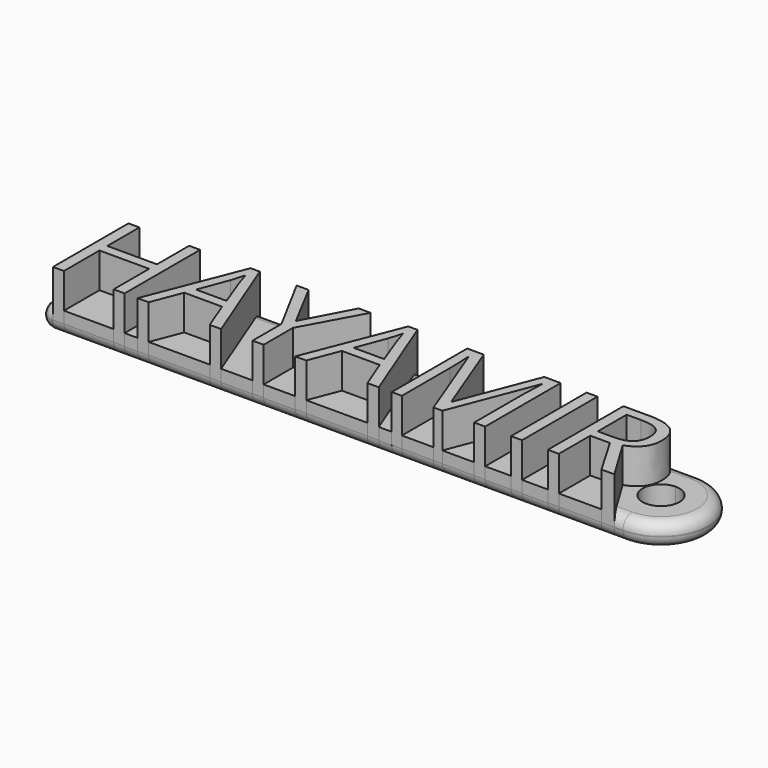
from build123d import *

# Parameters (mm, degrees)
F0_TEXT_SIZE   = 11.3354587318
F1_DEPTH       = 5
F0_W           = 4.2631951824
F0_H           = 3.8080056677
F2_DEPTH       = 2
F3_T1_DEPTH    = 5.9528869996
F3_T3_DEPTH    = 5.9741409848
F3_S1_T1_DEPTH = 5.9511158342
F3_S2_T1_DEPTH = 5.9528869996
F3_S2_T3_DEPTH = 5.9741409848
F3_S3_T1_DEPTH = 5.7580588027
F3_S3_T3_DEPTH = 5.9404888417
F3_S4_T1_DEPTH = 5.6597591215
F3_S5_T1_DEPTH = 5.6597591215
F3_S5_T3_DEPTH = 6.1122918881
F3_S6_T1_DEPTH = 5.9404888417
F3_2_T1_DEPTH  = 9.2631951824
F3_3_T1_DEPTH  = 48.9990343146
F3_3_T3_DEPTH  = 7.2240991066
F3_3_T5_DEPTH  = 7.2240991066
F3_3_T7_DEPTH  = 2.613740616
F3_3_T9_DEPTH  = 6.1118072185
F3_3_T11_DEPTH = 7.7005426064
F3_3_T13_DEPTH = 7.7058561027
F3_3_T15_DEPTH = 6.1595989161
F3_3_T17_DEPTH = 6.1171207148
F3_3_T19_DEPTH = 3.2374480655
F3_3_S23_W     = 1.1015022539
F3_3_S23_H     = 1.101502254
F3_3_T24_DEPTH = 1.101502254
F3_3_S29_W     = 1.1015022539
F3_3_S29_H     = 1.1015022539
F3_3_T30_DEPTH = 1.101502254
F3_3_S35_W     = 1.1015022539
F3_3_S35_H     = 1.1015022539
F3_3_T36_DEPTH = 1.101502254
F3_3_S41_W     = 1.1015022539
F3_3_S41_H     = 1.1015022539
F3_3_T42_DEPTH = 1.101502254
F3_3_T46_ANGLE = 180
F3_3_T48_ANGLE = 180
F3_4_T1_DEPTH  = 8.6486007793
F3_5_T1_DEPTH  = 7.7346794191
F3_6_T1_DEPTH  = 7.7116542685
F3_7_T1_DEPTH  = 10.2461919943
F3_8_T1_DEPTH  = 10.2461919943


# Not quite as in the source:
# - a fillet or chamfer that OpenCascade refuses, or shapes differently, is made with other operations: its cross-section is extruded or revolved along the edge and cut away or added
# - Text() gives the source's letters only with a copy of the font that has no kerning and outlines rounded to 1/6400 em; it was checked with that copy


with BuildPart() as f1:
    # F0 (on Top) → F1 (new body)
    with BuildSketch(Plane.XY):
        with Locations((-50, 0)):
            Text('HAYAMIR', F0_TEXT_SIZE, font='Open Sans', text_align=(TextAlign.LEFT, TextAlign.BOTTOM))
    extrude(amount=F1_DEPTH)

    # F3: fillet of radius 1 on 2 edges, made by hand

    # F3_s2 → F3_t1 (cut)
    with BuildSketch(Plane.YZ.offset(-44.1365568544)):
        with BuildLine():
            ThreePointArc((0, 1), (0.2928932188, 0.2928932188), (1, 0))
            Line((1, 0), (0, 0))
            Line((0, 0), (0, 1))
        make_face()
    extrude(amount=F3_T1_DEPTH, mode=Mode.SUBTRACT)

    # F3_s4 → F3_t3 (cut)
    with BuildSketch(Plane.YZ.offset(-37.9374778604)):
        with BuildLine():
            ThreePointArc((0, 1), (0.2928932188, 0.2928932188), (1, 0))
            Line((1, 0), (0, 0))
            Line((0, 0), (0, 1))
        make_face()
    extrude(amount=F3_T3_DEPTH, mode=Mode.SUBTRACT)

    # F3#s1: fillet of radius 1 on 1 edges, made by hand

    # F3_s1_s2 → F3_s1_t1 (cut)
    with BuildSketch(Plane.YZ.offset(-34.267623096)):
        with BuildLine():
            ThreePointArc((0, 1), (0.2928932188, 0.2928932188), (1, 0))
            Line((1, 0), (0, 0))
            Line((0, 0), (0, 1))
        make_face()
    extrude(amount=F3_S1_T1_DEPTH, mode=Mode.SUBTRACT)

    # F3#s2: fillet of radius 1 on 2 edges, made by hand

    # F3_s2_s2 → F3_s2_t1 (cut)
    with BuildSketch(Plane.YZ.offset(-30.6154799858)):
        with BuildLine():
            ThreePointArc((0, 1), (0.2928932188, 0.2928932188), (1, 0))
            Line((1, 0), (0, 0))
            Line((0, 0), (0, 1))
        make_face()
    extrude(amount=F3_S2_T1_DEPTH, mode=Mode.SUBTRACT)

    # F3_s2_s4 → F3_s2_t3 (cut)
    with BuildSketch(Plane.YZ.offset(-24.4164009919)):
        with BuildLine():
            ThreePointArc((0, 1), (0.2928932188, 0.2928932188), (1, 0))
            Line((1, 0), (0, 0))
            Line((0, 0), (0, 1))
        make_face()
    extrude(amount=F3_S2_T3_DEPTH, mode=Mode.SUBTRACT)

    # F3#s3: fillet of radius 1 on 3 edges, made by hand

    # F3_s3_s2 → F3_s3_t1 (cut)
    with BuildSketch(Plane.YZ.offset(-18.7486716259)):
        with BuildLine():
            ThreePointArc((0, 1), (0.2928932188, 0.2928932188), (1, 0))
            Line((1, 0), (0, 0))
            Line((0, 0), (0, 1))
        make_face()
    extrude(amount=F3_S3_T1_DEPTH, mode=Mode.SUBTRACT)

    # F3_s3_s4 → F3_s3_t3 (cut)
    with BuildSketch(Plane.YZ.offset(-15.2559334042)):
        with BuildLine():
            ThreePointArc((1, 0), (0.2928932188, 0.2928932188), (0, 1))
            Line((0, 1), (0, 0))
            Line((0, 0), (1, 0))
        make_face()
    extrude(amount=F3_S3_T3_DEPTH, mode=Mode.SUBTRACT)

    # F3#s4: fillet of radius 1 on 1 edges, made by hand

    # F3_s4_s2 → F3_s4_t1 (cut)
    with BuildSketch(Plane.YZ.offset(-11.8154445625)):
        with BuildLine():
            ThreePointArc((1, 0), (0.2928932188, 0.2928932188), (0, 1))
            Line((0, 1), (0, 0))
            Line((0, 0), (1, 0))
        make_face()
    extrude(amount=F3_S4_T1_DEPTH, mode=Mode.SUBTRACT)

    # F3#s5: fillet of radius 1 on 2 edges, made by hand

    # F3_s5_s2 → F3_s5_t1 (cut)
    with BuildSketch(Plane.YZ.offset(-8.655685441)):
        with BuildLine():
            ThreePointArc((1, 0), (0.2928932188, 0.2928932188), (0, 1))
            Line((0, 1), (0, 0))
            Line((0, 0), (1, 0))
        make_face()
    extrude(amount=F3_S5_T1_DEPTH, mode=Mode.SUBTRACT)

    # F3_s5_s4 → F3_s5_t3 (cut)
    with BuildSketch(Plane.YZ.offset(-4.3473255402)):
        with BuildLine():
            ThreePointArc((0, 1), (0.2928932188, 0.2928932188), (1, 0))
            Line((1, 0), (0, 0))
            Line((0, 0), (0, 1))
        make_face()
    extrude(amount=F3_S5_T3_DEPTH, mode=Mode.SUBTRACT)

    # F3#s6: fillet of radius 1 on 2 edges, made by hand

    # F3_s6_s2 → F3_s6_t1 (cut)
    with BuildSketch(Plane.YZ.offset(-51.3877081119)):
        with BuildLine():
            ThreePointArc((1, 0), (0.2928932188, 0.2928932188), (0, 1))
            Line((0, 1), (0, 0))
            Line((0, 0), (1, 0))
        make_face()
    extrude(amount=F3_S6_T1_DEPTH, mode=Mode.SUBTRACT)


with BuildPart() as f2:
    # F0 (on Top) → F2 (new body)
    with BuildSketch(Plane.XY):
        with Locations((-45.8156216791, 1.9040028339)):
            Rectangle(F0_W, F0_H)
    extrude(amount=F2_DEPTH)

    # F3#2: fillet of radius 1 on 1 edges, made by hand

    # F3_2_s2 → F3_2_t1 (cut)
    with BuildSketch(Plane.YZ.offset(-50.4472192703)):
        with BuildLine():
            ThreePointArc((0, 1), (0.2928932188, 0.2928932188), (1, 0))
            Line((1, 0), (0, 0))
            Line((0, 0), (0, 1))
        make_face()
    extrude(amount=F3_2_T1_DEPTH, mode=Mode.SUBTRACT)


with BuildPart() as f2b:
    # F0 (on Top) → F2, piece 2 (new body)
    with BuildSketch(Plane.XY):
        with BuildLine():
            ThreePointArc((0, 0), (4.0807651435, 4.0807651435), (0, 8.1615302869))
            Line((0, 8.1615302869), (0, 5.6615302869))
            ThreePointArc((0, 5.6615302869), (1.1177697524, 5.1985348959), (1.5807651435, 4.0807651435))
            ThreePointArc((1.5807651435, 4.0807651435), (1.1177697524, 2.9629953911), (0, 2.5))
            Line((0, 2.5), (0, 0))
        make_face()
        with BuildLine():
            Line((-50, 8.1615302869), (-50, 0))
            Line((-50, 0), (-48.8877081119, 0))
            Line((-48.8877081119, 0), (-48.8877081119, 8.0924548353))
            Line((-48.8877081119, 8.0924548353), (-47.9472192703, 8.0924548353))
            Line((-47.9472192703, 8.0924548353), (-47.9472192703, 4.6493092455))
            Line((-47.9472192703, 4.6493092455), (-43.6840240878, 4.6493092455))
            Line((-43.6840240878, 4.6493092455), (-43.6840240878, 8.0924548353))
            Line((-43.6840240878, 8.0924548353), (-42.7435352462, 8.0924548353))
            Line((-42.7435352462, 8.0924548353), (-42.7435352462, 0))
            Line((-42.7435352462, 0), (-41.6365568544, 0))
            Line((-41.6365568544, 0), (-38.4378320935, 8.1261069784))
            Line((-38.4378320935, 8.1261069784), (-37.6461211477, 8.1261069784))
            Line((-37.6461211477, 8.1261069784), (-34.4633368757, 0))
            Line((-34.4633368757, 0), (-31.767623096, 0))
            Line((-31.767623096, 0), (-31.767623096, 3.0942260007))
            Line((-31.767623096, 3.0942260007), (-34.4633368757, 8.0924548353))
            Line((-34.4633368757, 8.0924548353), (-33.4342897627, 8.0924548353))
            Line((-33.4342897627, 8.0924548353), (-31.2911795962, 4.0453418349))
            Line((-31.2911795962, 4.0453418349), (-29.1339001063, 8.0924548353))
            Line((-29.1339001063, 8.0924548353), (-28.1154799858, 8.0924548353))
            Line((-28.1154799858, 8.0924548353), (-30.8165072618, 3.1385051364))
            Line((-30.8165072618, 3.1385051364), (-30.8165072618, 0))
            Line((-30.8165072618, 0), (-28.1154799858, 0))
            Line((-28.1154799858, 0), (-24.9167552249, 8.1261069784))
            Line((-24.9167552249, 8.1261069784), (-24.1250442791, 8.1261069784))
            Line((-24.1250442791, 8.1261069784), (-20.9422600071, 0))
            Line((-20.9422600071, 0), (-19.829968119, 0))
            Line((-19.829968119, 0), (-19.829968119, 8.0924548353))
            Line((-19.829968119, 8.0924548353), (-18.4130357775, 8.0924548353))
            Line((-18.4130357775, 8.0924548353), (-15.8501594049, 1.4169323415))
            Line((-15.8501594049, 1.4169323415), (-15.8058802692, 1.4169323415))
            Line((-15.8058802692, 1.4169323415), (-13.2217499114, 8.0924548353))
            Line((-13.2217499114, 8.0924548353), (-11.8154445625, 8.0924548353))
            Line((-11.8154445625, 8.0924548353), (-11.8154445625, 0))
            Line((-11.8154445625, 0), (-9.5961742827, 0))
            Line((-9.5961742827, 0), (-9.5961742827, 8.0924548353))
            Line((-9.5961742827, 8.0924548353), (-8.655685441, 8.0924548353))
            Line((-8.655685441, 8.0924548353), (-8.655685441, 0))
            Line((-8.655685441, 0), (-6.4364151612, 0))
            Line((-6.4364151612, 0), (-6.4364151612, 8.0924548353))
            Line((-6.4364151612, 8.0924548353), (-4.2171448813, 8.0924548353))
            add(Edge.make_bspline(
                [(-4.2171448813, 8.0924548353), (-2.7275947574, 8.0924548353), (-2.0164718385, 7.5221395678)],
                knots=[0, 0, 0, 1, 1, 1], degree=2))
            add(Edge.make_bspline(
                [(-2.0164718385, 7.5221395678), (-1.3053489196, 6.9518243004), (-1.3053489196, 5.8058802692)],
                knots=[0, 0, 0, 1, 1, 1], degree=2))
            add(Edge.make_bspline(
                [(-1.3053489196, 5.8058802692), (-1.3053489196, 4.2012043925), (-2.9330499469, 3.6362026213)],
                knots=[0, 0, 0, 1, 1, 1], degree=2))
            Line((-2.9330499469, 3.6362026213), (-0.7350336521, 0))
            Line((-0.7350336521, 0), (0, 0))
            Line((0, 0), (0, 2.5))
            ThreePointArc((0, 2.5), (-1.5807651435, 4.0807651435), (0, 5.6615302869))
            Line((0, 5.6615302869), (0, 8.1615302869))
            Line((0, 8.1615302869), (-50, 8.1615302869))
        make_face()
    extrude(amount=F2_DEPTH)

    # F3#3: fillet of radius 1 on 18 edges, made by hand

    # F3_3_s2 → F3_3_t1 (cut)
    with BuildSketch(Plane.YZ.offset(-48.9990343146)):
        with BuildLine():
            ThreePointArc((8.1619302869, 0.9990343146), (7.8686370681, 1.7071067812), (7.1605646015, 2.0004))
            Line((7.1605646015, 2.0004), (7.1605646015, 2.1005365685))
            ThreePointArc((7.1605646015, 2.1005365685), (7.6610474442, 2.1001365685), (8.1615302869, 2.1001365685))
            Line((8.1615302869, 2.1001365685), (8.2616668555, 2))
            ThreePointArc((8.2616668555, 2), (8.2616668555, 1.4995171573), (8.2620668555, 0.9990343146))
            Line((8.2620668555, 0.9990343146), (8.1619302869, 0.9990343146))
        make_face()
        with BuildLine():
            ThreePointArc((8.1619302869, 1.0009656854), (7.8686370681, 0.2928932188), (7.1605646015, -0.0004))
            Line((7.1605646015, -0.0004), (7.1605646015, -0.1005365685))
            ThreePointArc((7.1605646015, -0.1005365685), (7.6610474442, -0.1001365685), (8.1615302869, -0.1001365685))
            Line((8.1615302869, -0.1001365685), (8.2616668555, 0))
            ThreePointArc((8.2616668555, 0), (8.2616668555, 0.5004828427), (8.2620668555, 1.0009656854))
            Line((8.2620668555, 1.0009656854), (8.1619302869, 1.0009656854))
        make_face()
    extrude(amount=F3_3_T1_DEPTH, mode=Mode.SUBTRACT)

    # F3_3_s4 → F3_3_t3 (cut)
    with BuildSketch(Plane.YZ.offset(-14.3178589759)):
        with BuildLine():
            ThreePointArc((-0.0004, 1.0009656854), (0.2928932188, 0.2928932188), (1.0009656854, -0.0004))
            Line((1.0009656854, -0.0004), (1.0009656854, -0.1005365685))
            ThreePointArc((1.0009656854, -0.1005365685), (0.5004828427, -0.1001365685), (0, -0.1001365685))
            Line((0, -0.1001365685), (-0.1001365685, 0))
            ThreePointArc((-0.1001365685, 0), (-0.1001365685, 0.5004828427), (-0.1005365685, 1.0009656854))
            Line((-0.1005365685, 1.0009656854), (-0.0004, 1.0009656854))
        make_face()
    extrude(amount=F3_3_T3_DEPTH, mode=Mode.SUBTRACT)

    # F3_3_s6 → F3_3_t5 (cut)
    with BuildSketch(Plane.YZ.offset(-11.1580998544)):
        with BuildLine():
            ThreePointArc((-0.0004, 1.0009656854), (0.2928932188, 0.2928932188), (1.0009656854, -0.0004))
            Line((1.0009656854, -0.0004), (1.0009656854, -0.1005365685))
            ThreePointArc((1.0009656854, -0.1005365685), (0.5004828427, -0.1001365685), (0, -0.1001365685))
            Line((0, -0.1001365685), (-0.1001365685, 0))
            ThreePointArc((-0.1001365685, 0), (-0.1001365685, 0.5004828427), (-0.1005365685, 1.0009656854))
            Line((-0.1005365685, 1.0009656854), (-0.0004, 1.0009656854))
        make_face()
    extrude(amount=F3_3_T5_DEPTH, mode=Mode.SUBTRACT)

    # F3_3_s8 → F3_3_t7 (cut)
    with BuildSketch(Plane.YZ.offset(-48.9990343146)):
        with BuildLine():
            ThreePointArc((-0.0004, 1.0009656854), (0.2928932188, 0.2928932188), (1.0009656854, -0.0004))
            Line((1.0009656854, -0.0004), (1.0009656854, -0.1005365685))
            ThreePointArc((1.0009656854, -0.1005365685), (0.5004828427, -0.1001365685), (0, -0.1001365685))
            Line((0, -0.1001365685), (-0.1001365685, 0))
            ThreePointArc((-0.1001365685, 0), (-0.1001365685, 0.5004828427), (-0.1005365685, 1.0009656854))
            Line((-0.1005365685, 1.0009656854), (-0.0004, 1.0009656854))
        make_face()
        with BuildLine():
            ThreePointArc((-0.0004, 0.9990343146), (0.2928932188, 1.7071067812), (1.0009656854, 2.0004))
            Line((1.0009656854, 2.0004), (1.0009656854, 2.1005365685))
            ThreePointArc((1.0009656854, 2.1005365685), (0.5004828427, 2.1001365685), (0, 2.1001365685))
            Line((0, 2.1001365685), (-0.1001365685, 2))
            ThreePointArc((-0.1001365685, 2), (-0.1001365685, 1.4995171573), (-0.1005365685, 0.9990343146))
            Line((-0.1005365685, 0.9990343146), (-0.0004, 0.9990343146))
        make_face()
    extrude(amount=F3_3_T7_DEPTH, mode=Mode.SUBTRACT)

    # F3_3_s10 → F3_3_t9 (cut)
    with BuildSketch(Plane.YZ.offset(-45.2459496596)):
        with BuildLine():
            ThreePointArc((-0.0004, 1.0009656854), (0.2928932188, 0.2928932188), (1.0009656854, -0.0004))
            Line((1.0009656854, -0.0004), (1.0009656854, -0.1005365685))
            ThreePointArc((1.0009656854, -0.1005365685), (0.5004828427, -0.1001365685), (0, -0.1001365685))
            Line((0, -0.1001365685), (-0.1001365685, 0))
            ThreePointArc((-0.1001365685, 0), (-0.1001365685, 0.5004828427), (-0.1005365685, 1.0009656854))
            Line((-0.1005365685, 1.0009656854), (-0.0004, 1.0009656854))
        make_face()
    extrude(amount=F3_3_T9_DEPTH, mode=Mode.SUBTRACT)

    # F3_3_s12 → F3_3_t11 (cut)
    with BuildSketch(Plane.YZ.offset(-36.965751289)):
        with BuildLine():
            ThreePointArc((-0.0004, 1.0009656854), (0.2928932188, 0.2928932188), (1.0009656854, -0.0004))
            Line((1.0009656854, -0.0004), (1.0009656854, -0.1005365685))
            ThreePointArc((1.0009656854, -0.1005365685), (0.5004828427, -0.1001365685), (0, -0.1001365685))
            Line((0, -0.1001365685), (-0.1001365685, 0))
            ThreePointArc((-0.1001365685, 0), (-0.1001365685, 0.5004828427), (-0.1005365685, 1.0009656854))
            Line((-0.1005365685, 1.0009656854), (-0.0004, 1.0009656854))
        make_face()
    extrude(amount=F3_3_T11_DEPTH, mode=Mode.SUBTRACT)

    # F3_3_s14 → F3_3_t13 (cut)
    with BuildSketch(Plane.YZ.offset(-33.3189216751)):
        with BuildLine():
            ThreePointArc((-0.0004, 1.0009656854), (0.2928932188, 0.2928932188), (1.0009656854, -0.0004))
            Line((1.0009656854, -0.0004), (1.0009656854, -0.1005365685))
            ThreePointArc((1.0009656854, -0.1005365685), (0.5004828427, -0.1001365685), (0, -0.1001365685))
            Line((0, -0.1001365685), (-0.1001365685, 0))
            ThreePointArc((-0.1001365685, 0), (-0.1001365685, 0.5004828427), (-0.1005365685, 1.0009656854))
            Line((-0.1005365685, 1.0009656854), (-0.0004, 1.0009656854))
        make_face()
    extrude(amount=F3_3_T13_DEPTH, mode=Mode.SUBTRACT)

    # F3_3_s16 → F3_3_t15 (cut)
    with BuildSketch(Plane.XZ.offset(-7.1605646015)):
        with BuildLine():
            ThreePointArc((-50.0004, 1.0009656854), (-49.7071067812, 0.2928932188), (-48.9990343146, -0.0004))
            Line((-48.9990343146, -0.0004), (-48.9990343146, -0.1005365685))
            ThreePointArc((-48.9990343146, -0.1005365685), (-49.4995171573, -0.1001365685), (-50, -0.1001365685))
            Line((-50, -0.1001365685), (-50.1001365685, 0))
            ThreePointArc((-50.1001365685, 0), (-50.1001365685, 0.5004828427), (-50.1005365685, 1.0009656854))
            Line((-50.1005365685, 1.0009656854), (-50.0004, 1.0009656854))
        make_face()
        with BuildLine():
            ThreePointArc((-50.0004, 0.9990343146), (-49.7071067812, 1.7071067812), (-48.9990343146, 2.0004))
            Line((-48.9990343146, 2.0004), (-48.9990343146, 2.1005365685))
            ThreePointArc((-48.9990343146, 2.1005365685), (-49.4995171573, 2.1001365685), (-50, 2.1001365685))
            Line((-50, 2.1001365685), (-50.1001365685, 2))
            ThreePointArc((-50.1001365685, 2), (-50.1001365685, 1.4995171573), (-50.1005365685, 0.9990343146))
            Line((-50.1005365685, 0.9990343146), (-50.0004, 0.9990343146))
        make_face()
    extrude(amount=F3_3_T15_DEPTH, mode=Mode.SUBTRACT)

    # F3_3_s18 → F3_3_t17 (cut)
    with BuildSketch(Plane.YZ.offset(-23.4446744205)):
        with BuildLine():
            ThreePointArc((-0.0004, 1.0009656854), (0.2928932188, 0.2928932188), (1.0009656854, -0.0004))
            Line((1.0009656854, -0.0004), (1.0009656854, -0.1005365685))
            ThreePointArc((1.0009656854, -0.1005365685), (0.5004828427, -0.1001365685), (0, -0.1001365685))
            Line((0, -0.1001365685), (-0.1001365685, 0))
            ThreePointArc((-0.1001365685, 0), (-0.1001365685, 0.5004828427), (-0.1005365685, 1.0009656854))
            Line((-0.1005365685, 1.0009656854), (-0.0004, 1.0009656854))
        make_face()
    extrude(amount=F3_3_T17_DEPTH, mode=Mode.SUBTRACT)

    # F3_3_s20 → F3_3_t19 (cut)
    with BuildSketch(Plane.YZ.offset(-3.2374480655)):
        with BuildLine():
            ThreePointArc((-0.0004, 1.0009656854), (0.2928932188, 0.2928932188), (1.0009656854, -0.0004))
            Line((1.0009656854, -0.0004), (1.0009656854, -0.1005365685))
            ThreePointArc((1.0009656854, -0.1005365685), (0.5004828427, -0.1001365685), (0, -0.1001365685))
            Line((0, -0.1001365685), (-0.1001365685, 0))
            ThreePointArc((-0.1001365685, 0), (-0.1001365685, 0.5004828427), (-0.1005365685, 1.0009656854))
            Line((-0.1005365685, 1.0009656854), (-0.0004, 1.0009656854))
        make_face()
        with BuildLine():
            ThreePointArc((-0.0004, 0.9990343146), (0.2928932188, 1.7071067812), (1.0009656854, 2.0004))
            Line((1.0009656854, 2.0004), (1.0009656854, 2.1005365685))
            ThreePointArc((1.0009656854, 2.1005365685), (0.5004828427, 2.1001365685), (0, 2.1001365685))
            Line((0, 2.1001365685), (-0.1001365685, 2))
            ThreePointArc((-0.1001365685, 2), (-0.1001365685, 1.4995171573), (-0.1005365685, 0.9990343146))
            Line((-0.1005365685, 0.9990343146), (-0.0004, 0.9990343146))
        make_face()
    extrude(amount=F3_3_T19_DEPTH, mode=Mode.SUBTRACT)


with BuildPart() as f2c:
    # F0 (on Top) → F2, piece 3 (new body)
    with BuildSketch(Plane.XY):
        with BuildLine():
            Line((-5.4959263195, 7.2670917464), (-5.4959263195, 4.1728657457))
            Line((-5.4959263195, 4.1728657457), (-4.2047467233, 4.1728657457))
            add(Edge.make_bspline(
                [(-4.2047467233, 4.1728657457), (-3.2093517535, 4.1728657457), (-2.7444208289, 4.5687212186)],
                knots=[0, 0, 0, 1, 1, 1], degree=2))
            add(Edge.make_bspline(
                [(-2.7444208289, 4.5687212186), (-2.2794899044, 4.9645766915), (-2.2794899044, 5.7562876373)],
                knots=[0, 0, 0, 1, 1, 1], degree=2))
            add(Edge.make_bspline(
                [(-2.2794899044, 5.7562876373), (-2.2794899044, 6.5586255756), (-2.7523910733, 6.912858661)],
                knots=[0, 0, 0, 1, 1, 1], degree=2))
            add(Edge.make_bspline(
                [(-2.7523910733, 6.912858661), (-3.2252922423, 7.2670917464), (-4.2720510096, 7.2670917464)],
                knots=[0, 0, 0, 1, 1, 1], degree=2))
            Line((-4.2720510096, 7.2670917464), (-5.4959263195, 7.2670917464))
        make_face()
    extrude(amount=F2_DEPTH)


with BuildPart() as f2d:
    # F0 (on Top) → F2, piece 4 (new body)
    with BuildSketch(Plane.XY):
        Polygon((-5.4959263195, 0), (-1.8473255402, 0), (-3.8062345023, 3.365214311), (-5.4959263195, 3.365214311), align=None)
    extrude(amount=F2_DEPTH)

    # F3#4: fillet of radius 1 on 1 edges, made by hand

    # F3_4_s2 → F3_4_t1 (cut)
    with BuildSketch(Plane.YZ.offset(-7.9959263195)):
        with BuildLine():
            ThreePointArc((0, 1), (0.2928932188, 0.2928932188), (1, 0))
            Line((1, 0), (0, 0))
            Line((0, 0), (0, 1))
        make_face()
    extrude(amount=F3_4_T1_DEPTH, mode=Mode.SUBTRACT)


with BuildPart() as f2e:
    # F0 (on Top) → F2, piece 5 (new body)
    with BuildSketch(Plane.XY):
        with BuildLine():
            Line((-15.4906128232, 0), (-12.7559334042, 0))
            Line((-12.7559334042, 0), (-12.7559334042, 5.2143110166))
            add(Edge.make_bspline(
                [(-12.7559334042, 5.2143110166), (-12.7559334042, 6.1105207226), (-12.6780021254, 7.1625929862)],
                knots=[0, 0, 0, 1, 1, 1], degree=2))
            Line((-12.6780021254, 7.1625929862), (-12.7222812611, 7.1625929862))
            Line((-12.7222812611, 7.1625929862), (-15.4906128232, 0))
        make_face()
    extrude(amount=F2_DEPTH)

    # F3#5: fillet of radius 1 on 1 edges, made by hand

    # F3_5_s2 → F3_5_t1 (cut)
    with BuildSketch(Plane.YZ.offset(-17.9906128232)):
        with BuildLine():
            ThreePointArc((0, 1), (0.2928932188, 0.2928932188), (1, 0))
            Line((1, 0), (0, 0))
            Line((0, 0), (0, 1))
        make_face()
    extrude(amount=F3_5_T1_DEPTH, mode=Mode.SUBTRACT)


with BuildPart() as f2f:
    # F0 (on Top) → F2, piece 6 (new body)
    with BuildSketch(Plane.XY):
        with BuildLine():
            Line((-18.9603258944, 0), (-16.2486716259, 0))
            Line((-16.2486716259, 0), (-18.9939780375, 7.1732199787))
            Line((-18.9939780375, 7.1732199787), (-19.0382571732, 7.1732199787))
            add(Edge.make_bspline(
                [(-19.0382571732, 7.1732199787), (-18.9603258944, 6.3212894084), (-18.9603258944, 5.1470067304)],
                knots=[0, 0, 0, 1, 1, 1], degree=2))
            Line((-18.9603258944, 5.1470067304), (-18.9603258944, 0))
        make_face()
    extrude(amount=F2_DEPTH)

    # F3#6: fillet of radius 1 on 1 edges, made by hand

    # F3_6_s2 → F3_6_t1 (cut)
    with BuildSketch(Plane.YZ.offset(-21.4603258944)):
        with BuildLine():
            ThreePointArc((0, 1), (0.2928932188, 0.2928932188), (1, 0))
            Line((1, 0), (0, 0))
            Line((0, 0), (0, 1))
        make_face()
    extrude(amount=F3_6_T1_DEPTH, mode=Mode.SUBTRACT)


with BuildPart() as f2g:
    # F0 (on Top) → F2, piece 7 (new body)
    with BuildSketch(Plane.XY):
        Polygon((-26.1671980163, 2.5735033652), (-27.1625929862, 0), (-21.9164009919, 0), (-22.9241941197, 2.5735033652), align=None)
    extrude(amount=F2_DEPTH)

    # F3#7: fillet of radius 1 on 1 edges, made by hand

    # F3_7_s2 → F3_7_t1 (cut)
    with BuildSketch(Plane.YZ.offset(-29.6625929862)):
        with BuildLine():
            ThreePointArc((0, 1), (0.2928932188, 0.2928932188), (1, 0))
            Line((1, 0), (0, 0))
            Line((0, 0), (0, 1))
        make_face()
    extrude(amount=F3_7_T1_DEPTH, mode=Mode.SUBTRACT)


with BuildPart() as f2h:
    # F0 (on Top) → F2, piece 8 (new body)
    with BuildSketch(Plane.XY):
        with BuildLine():
            Line((-25.834218916, 3.4201204392), (-23.2164364152, 3.4201204392))
            Line((-23.2164364152, 3.4201204392), (-24.1586964222, 5.9280906837))
            add(Edge.make_bspline(
                [(-24.1586964222, 5.9280906837), (-24.3411264612, 6.4045341835), (-24.5341834927, 7.0952887)],
                knots=[0, 0, 0, 1, 1, 1], degree=2))
            add(Edge.make_bspline(
                [(-24.5341834927, 7.0952887), (-24.6563939072, 6.5639390719), (-24.8831030818, 5.9280906837)],
                knots=[0, 0, 0, 1, 1, 1], degree=2))
            Line((-24.8831030818, 5.9280906837), (-25.834218916, 3.4201204392))
        make_face()
    extrude(amount=F2_DEPTH)


with BuildPart() as f2i:
    # F0 (on Top) → F2, piece 9 (new body)
    with BuildSketch(Plane.XY):
        Polygon((-39.6882748849, 2.5735033652), (-40.6836698548, 0), (-35.4374778604, 0), (-36.4452709883, 2.5735033652), align=None)
    extrude(amount=F2_DEPTH)

    # F3#8: fillet of radius 1 on 1 edges, made by hand

    # F3_8_s2 → F3_8_t1 (cut)
    with BuildSketch(Plane.YZ.offset(-43.1836698548)):
        with BuildLine():
            ThreePointArc((0, 1), (0.2928932188, 0.2928932188), (1, 0))
            Line((1, 0), (0, 0))
            Line((0, 0), (0, 1))
        make_face()
    extrude(amount=F3_8_T1_DEPTH, mode=Mode.SUBTRACT)


with BuildPart() as f2j:
    # F0 (on Top) → F2, piece 10 (new body)
    with BuildSketch(Plane.XY):
        with BuildLine():
            Line((-39.3552957846, 3.4201204392), (-36.7375132837, 3.4201204392))
            Line((-36.7375132837, 3.4201204392), (-37.6797732908, 5.9280906837))
            add(Edge.make_bspline(
                [(-37.6797732908, 5.9280906837), (-37.8622033298, 6.4045341835), (-38.0552603613, 7.0952887)],
                knots=[0, 0, 0, 1, 1, 1], degree=2))
            add(Edge.make_bspline(
                [(-38.0552603613, 7.0952887), (-38.1774707758, 6.5639390719), (-38.4041799504, 5.9280906837)],
                knots=[0, 0, 0, 1, 1, 1], degree=2))
            Line((-38.4041799504, 5.9280906837), (-39.3552957846, 3.4201204392))
        make_face()
    extrude(amount=F2_DEPTH)


with BuildPart() as f3_3_tool22:
    # F3_3_s23 → F3_3_t24 (new body)
    with BuildSketch(Plane.XY.offset(0.9990343146)):
        with Locations((-49.5497854416, 7.7113157285)):
            Rectangle(F3_3_S23_W, F3_3_S23_H)
    extrude(amount=F3_3_T24_DEPTH)

    # F3_3_s25 → F3_3_t26 (revolve, cut)
    with BuildSketch(Plane(origin=(-48.9990343146, 7.1605646015, 0.9990343146), x_dir=(0.7071067812, -0.7071067812, 0), z_dir=(-0.7071067812, -0.7071067812, 0))):
        with BuildLine():
            ThreePointArc((0, -1.0013656854), (1.0013656854, 0), (0, 1.0013656854))
            Line((0, 1.0013656854), (0, -1.0013656854))
        make_face()
    revolve(axis=Axis((-48.9990343146, 7.1605646015, 0.9990343146), (0, 0, 1)), mode=Mode.SUBTRACT)


with BuildPart() as f2b_1:
    add(f2b.part)

    # F3_3_t21: cut F3_3_tool22
    add(f3_3_tool22.part, mode=Mode.SUBTRACT)


with BuildPart() as f3_3_tool28:
    # F3_3_s29 → F3_3_t30 (new body)
    with BuildSketch(Plane.XZ.offset(-7.1605646015)):
        with Locations((-49.5497854416, 0.4502145584)):
            Rectangle(F3_3_S29_W, F3_3_S29_H)
    extrude(amount=-F3_3_T30_DEPTH)

    # F3_3_s31 → F3_3_t32 (revolve, cut)
    with BuildSketch(Plane(origin=(-48.9990343146, 7.1605646015, 1.0009656854), x_dir=(0.7071067812, 0, 0.7071067812), z_dir=(-0.7071067812, 0, 0.7071067812))):
        with BuildLine():
            ThreePointArc((0, -1.0013656854), (1.0013656854, 0), (0, 1.0013656854))
            Line((0, 1.0013656854), (0, -1.0013656854))
        make_face()
    revolve(axis=Axis((-48.9990343146, 7.1605646015, 1.0009656854), (0, 1, 0)), mode=Mode.SUBTRACT)


with BuildPart() as f2b_2:
    add(f2b_1.part)

    # F3_3_t27: cut F3_3_tool28
    add(f3_3_tool28.part, mode=Mode.SUBTRACT)


with BuildPart() as f3_3_tool34:
    # F3_3_s35 → F3_3_t36 (new body)
    with BuildSketch(Plane.YZ.offset(-48.9990343146)):
        with Locations((0.4502145584, 0.4502145584)):
            Rectangle(F3_3_S35_W, F3_3_S35_H)
    extrude(amount=-F3_3_T36_DEPTH)

    # F3_3_s37 → F3_3_t38 (revolve, cut)
    with BuildSketch(Plane(origin=(-48.9990343146, 1.0009656854, 1.0009656854), x_dir=(0, 0.7071067812, 0.7071067812), z_dir=(0, -0.7071067812, 0.7071067812))):
        with BuildLine():
            ThreePointArc((0, -1.0013656854), (1.0013656854, 0), (0, 1.0013656854))
            Line((0, 1.0013656854), (0, -1.0013656854))
        make_face()
    revolve(axis=Axis((-48.9990343146, 1.0009656854, 1.0009656854), (-1, 0, 0)), mode=Mode.SUBTRACT)


with BuildPart() as f2b_3:
    add(f2b_2.part)

    # F3_3_t33: cut F3_3_tool34
    add(f3_3_tool34.part, mode=Mode.SUBTRACT)


with BuildPart() as f3_3_tool40:
    # F3_3_s41 → F3_3_t42 (new body)
    with BuildSketch(Plane.XY.offset(0.9990343146)):
        with Locations((-49.5497854416, 0.4502145584)):
            Rectangle(F3_3_S41_W, F3_3_S41_H)
    extrude(amount=F3_3_T42_DEPTH)

    # F3_3_s43 → F3_3_t44 (revolve, cut)
    with BuildSketch(Plane(origin=(-48.9990343146, 1.0009656854, 0.9990343146), x_dir=(0.7071067812, 0.7071067812, 0), z_dir=(0.7071067812, -0.7071067812, 0))):
        with BuildLine():
            ThreePointArc((0, -1.0013656854), (1.0013656854, 0), (0, 1.0013656854))
            Line((0, 1.0013656854), (0, -1.0013656854))
        make_face()
    revolve(axis=Axis((-48.9990343146, 1.0009656854, 0.9990343146), (0, 0, 1)), mode=Mode.SUBTRACT)


with BuildPart() as f2b_4:
    add(f2b_3.part)

    # F3_3_t39: cut F3_3_tool40
    add(f3_3_tool40.part, mode=Mode.SUBTRACT)

    # F3_3_s45 → F3_3_t46 (revolve, cut)
    with BuildSketch(Plane.YZ):
        with BuildLine():
            ThreePointArc((-0.0004, 1.0009656854), (0.2928932188, 0.2928932188), (1.0009656854, -0.0004))
            Line((1.0009656854, -0.0004), (1.0009656854, -0.1005365685))
            ThreePointArc((1.0009656854, -0.1005365685), (0.5004828427, -0.1001365685), (0, -0.1001365685))
            Line((0, -0.1001365685), (-0.1001365685, 0))
            ThreePointArc((-0.1001365685, 0), (-0.1001365685, 0.5004828427), (-0.1005365685, 1.0009656854))
            Line((-0.1005365685, 1.0009656854), (-0.0004, 1.0009656854))
        make_face()
    revolve(axis=Axis((0, 4.0807651435, 0), (0, 0, 1)), revolution_arc=F3_3_T46_ANGLE, mode=Mode.SUBTRACT)

    # F3_3_s47 → F3_3_t48 (revolve, cut)
    with BuildSketch(Plane.YZ):
        with BuildLine():
            ThreePointArc((-0.0004, 0.9990343146), (0.2928932188, 1.7071067812), (1.0009656854, 2.0004))
            Line((1.0009656854, 2.0004), (1.0009656854, 2.1005365685))
            ThreePointArc((1.0009656854, 2.1005365685), (0.5004828427, 2.1001365685), (0, 2.1001365685))
            Line((0, 2.1001365685), (-0.1001365685, 2))
            ThreePointArc((-0.1001365685, 2), (-0.1001365685, 1.4995171573), (-0.1005365685, 0.9990343146))
            Line((-0.1005365685, 0.9990343146), (-0.0004, 0.9990343146))
        make_face()
    revolve(axis=Axis((0, 4.0807651435, 2), (0, 0, 1)), revolution_arc=F3_3_T48_ANGLE, mode=Mode.SUBTRACT)


solid = Compound([f1.part, f2.part, f2c.part, f2d.part, f2e.part, f2f.part, f2g.part, f2h.part, f2i.part, f2j.part, f2b_4.part])
